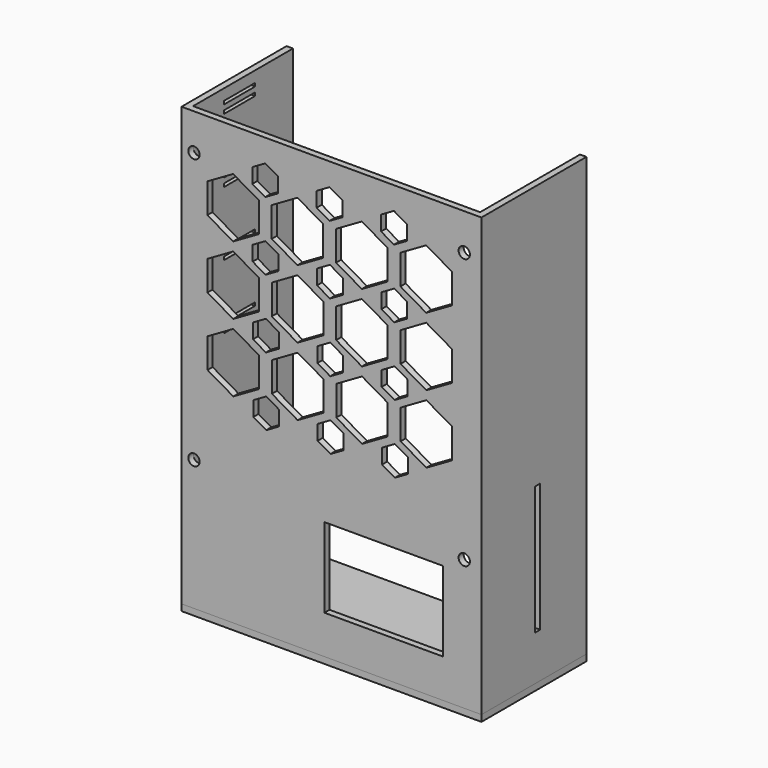
from build123d import *

# Parameters (mm, degrees)
F1_DEPTH  = 170
F2_W      = 116.5
F2_H      = 2.5
F3_DEPTH  = 51
F4_W      = 46
F4_H      = 31
F5_DEPTH  = 10
F7_DEPTH  = 25
F9_D      = 11
F9_DEPTH  = 38.5365562692
F11_DEPTH = 25
F13_D     = 4.4
F14_W     = 15
F14_H     = 1.25
F15_DEPTH = 51
F16_W     = 2.5
F16_H     = 50
F17_DEPTH = 80


# Not quite as in the source:
# - a feature names something its author has since deleted; it is built from what else it names


with BuildPart() as f1:
    # F0 (on Top) → F1 (new body)
    with BuildSketch(Plane.XY):
        Polygon((-38.5355562692, 51), (-38.5355562692, 0), (77.9644437308, 0), (77.9644437308, 51), (75.4644437308, 51), (75.4644437308, 2.4839404983), (-36.0355562692, 2.4839404983), (-36.0355562692, 51), align=None)
    extrude(amount=F1_DEPTH)

    # F4 (on Front) → F5 (cut)
    with BuildSketch(Plane.XZ):
        with Locations((39.9644437308, 30.5)):
            Rectangle(F4_W, F4_H)
    extrude(amount=-F5_DEPTH, mode=Mode.SUBTRACT)

    # F6 (on Front) → F7 (cut)
    with BuildSketch(Plane.XZ):
        Polygon((21.5, 136.2), (31.5, 130.4264973081), (41.5, 136.2), (41.5, 147.7470053838), (31.5, 153.5205080757), (21.5, 147.7470053838), align=None)
        Polygon((25.8301270189, 145.2470053838), (31.5, 148.5205080757), (37.1698729811, 145.2470053838), (37.1698729811, 138.7), (31.5, 135.4264973081), (25.8301270189, 138.7), align=None, mode=Mode.SUBTRACT)
        Polygon((56.5355562692, 127.0410161514), (46.5355562692, 121.2675134595), (46.5355562692, 109.7205080757), (56.5355562692, 103.9470053838), (66.5355562692, 109.7205080757), (66.5355562692, 121.2675134595), align=None)
        Polygon((56.5355562692, 108.9470053838), (50.8656832881, 112.2205080757), (50.8656832881, 118.7675134595), (56.5355562692, 122.0410161514), (62.2054292503, 118.7675134595), (62.2054292503, 112.2205080757), align=None, mode=Mode.SUBTRACT)
        Polygon((-3.4644437308, 121.2675134595), (-3.4644437308, 109.7205080757), (6.5355562692, 103.9470053838), (16.5355562692, 109.7205080757), (16.5355562692, 121.2675134595), (6.5355562692, 127.0410161514), align=None)
        Polygon((6.5355562692, 122.0410161514), (12.2054292503, 118.7675134595), (12.2054292503, 112.2205080757), (6.5355562692, 108.9470053838), (0.8656832881, 112.2205080757), (0.8656832881, 118.7675134595), align=None, mode=Mode.SUBTRACT)
        Polygon((21.5711125384, 83.2410161514), (31.5711125384, 77.4675134595), (41.5711125384, 83.2410161514), (41.5711125384, 94.7880215352), (31.5711125384, 100.5615242271), (21.5711125384, 94.7880215352), align=None)
        Polygon((25.9012395573, 92.2880215352), (31.5711125384, 95.5615242271), (37.2409855194, 92.2880215352), (37.2409855194, 85.7410161514), (31.5711125384, 82.4675134595), (25.9012395573, 85.7410161514), align=None, mode=Mode.SUBTRACT)
        Polygon((21.5355562692, 109.7205080757), (31.5355562692, 103.9470053838), (41.5355562692, 109.7205080757), (41.5355562692, 121.2675134595), (31.5355562692, 127.0410161514), (21.5355562692, 121.2675134595), align=None)
        Polygon((25.8656832881, 118.7675134595), (31.5355562692, 122.0410161514), (37.2054292503, 118.7675134595), (37.2054292503, 112.2205080757), (31.5355562692, 108.9470053838), (25.8656832881, 112.2205080757), align=None, mode=Mode.SUBTRACT)
        Polygon((-28.5, 147.7470053838), (-28.5, 136.2), (-18.5, 130.4264973081), (-8.5, 136.2), (-8.5, 147.7470053838), (-18.5, 153.5205080757), align=None)
        Polygon((-18.5, 135.4264973081), (-24.1698729811, 138.7), (-24.1698729811, 145.2470053838), (-18.5, 148.5205080757), (-12.8301270189, 145.2470053838), (-12.8301270189, 138.7), align=None, mode=Mode.SUBTRACT)
        Polygon((-28.4644437308, 121.2675134595), (-28.4644437308, 109.7205080757), (-18.4644437308, 103.9470053838), (-8.4644437308, 109.7205080757), (-8.4644437308, 121.2675134595), (-18.4644437308, 127.0410161514), align=None)
        Polygon((-18.4644437308, 108.9470053838), (-24.1343167119, 112.2205080757), (-24.1343167119, 118.7675134595), (-18.4644437308, 122.0410161514), (-12.7945707497, 118.7675134595), (-12.7945707497, 112.2205080757), align=None, mode=Mode.SUBTRACT)
        Polygon((-28.4288874616, 94.7880215352), (-28.4288874616, 83.2410161514), (-18.4288874616, 77.4675134595), (-8.4288874616, 83.2410161514), (-8.4288874616, 94.7880215352), (-18.4288874616, 100.5615242271), align=None)
        Polygon((-18.4288874616, 82.4675134595), (-24.0987604427, 85.7410161514), (-24.0987604427, 92.2880215352), (-18.4288874616, 95.5615242271), (-12.7590144806, 92.2880215352), (-12.7590144806, 85.7410161514), align=None, mode=Mode.SUBTRACT)
        Polygon((-3.4288874616, 94.7880215352), (-3.4288874616, 83.2410161514), (6.5711125384, 77.4675134595), (16.5711125384, 83.2410161514), (16.5711125384, 94.7880215352), (6.5711125384, 100.5615242271), align=None)
        Polygon((6.5711125384, 95.5615242271), (12.2409855194, 92.2880215352), (12.2409855194, 85.7410161514), (6.5711125384, 82.4675134595), (0.9012395573, 85.7410161514), (0.9012395573, 92.2880215352), align=None, mode=Mode.SUBTRACT)
        Polygon((56.5711125384, 100.5615242271), (46.5711125384, 94.7880215352), (46.5711125384, 83.2410161514), (56.5711125384, 77.4675134595), (66.5711125384, 83.2410161514), (66.5711125384, 94.7880215352), align=None)
        Polygon((56.5711125384, 82.4675134595), (50.9012395573, 85.7410161514), (50.9012395573, 92.2880215352), (56.5711125384, 95.5615242271), (62.2409855194, 92.2880215352), (62.2409855194, 85.7410161514), align=None, mode=Mode.SUBTRACT)
        Polygon((56.5, 153.5205080757), (46.5, 147.7470053838), (46.5, 136.2), (56.5, 130.4264973081), (66.5, 136.2), (66.5, 147.7470053838), align=None)
        Polygon((56.5, 135.4264973081), (50.8301270189, 138.7), (50.8301270189, 145.2470053838), (56.5, 148.5205080757), (62.1698729811, 145.2470053838), (62.1698729811, 138.7), align=None, mode=Mode.SUBTRACT)
        Polygon((-3.5, 147.7470053838), (-3.5, 136.2), (6.5, 130.4264973081), (16.5, 136.2), (16.5, 147.7470053838), (6.5, 153.5205080757), align=None)
        Polygon((6.5, 148.5205080757), (12.1698729811, 145.2470053838), (12.1698729811, 138.7), (6.5, 135.4264973081), (0.8301270189, 138.7), (0.8301270189, 145.2470053838), align=None, mode=Mode.SUBTRACT)
        Polygon((50.8301270189, 145.2470053838), (50.8301270189, 138.7), (56.5, 135.4264973081), (62.1698729811, 138.7), (62.1698729811, 145.2470053838), (56.5, 148.5205080757), align=None)
        Polygon((37.1698729811, 145.2470053838), (31.5, 148.5205080757), (25.8301270189, 145.2470053838), (25.8301270189, 138.7), (31.5, 135.4264973081), (37.1698729811, 138.7), align=None)
        Polygon((12.1698729811, 138.7), (12.1698729811, 145.2470053838), (6.5, 148.5205080757), (0.8301270189, 145.2470053838), (0.8301270189, 138.7), (6.5, 135.4264973081), align=None)
        Polygon((-24.1698729811, 145.2470053838), (-24.1698729811, 138.7), (-18.5, 135.4264973081), (-12.8301270189, 138.7), (-12.8301270189, 145.2470053838), (-18.5, 148.5205080757), align=None)
        Polygon((-24.1343167119, 118.7675134595), (-24.1343167119, 112.2205080757), (-18.4644437308, 108.9470053838), (-12.7945707497, 112.2205080757), (-12.7945707497, 118.7675134595), (-18.4644437308, 122.0410161514), align=None)
        Polygon((12.2054292503, 112.2205080757), (12.2054292503, 118.7675134595), (6.5355562692, 122.0410161514), (0.8656832881, 118.7675134595), (0.8656832881, 112.2205080757), (6.5355562692, 108.9470053838), align=None)
        Polygon((37.2054292503, 118.7675134595), (31.5355562692, 122.0410161514), (25.8656832881, 118.7675134595), (25.8656832881, 112.2205080757), (31.5355562692, 108.9470053838), (37.2054292503, 112.2205080757), align=None)
        Polygon((50.8656832881, 118.7675134595), (50.8656832881, 112.2205080757), (56.5355562692, 108.9470053838), (62.2054292503, 112.2205080757), (62.2054292503, 118.7675134595), (56.5355562692, 122.0410161514), align=None)
        Polygon((50.9012395573, 92.2880215352), (50.9012395573, 85.7410161514), (56.5711125384, 82.4675134595), (62.2409855194, 85.7410161514), (62.2409855194, 92.2880215352), (56.5711125384, 95.5615242271), align=None)
        Polygon((37.2409855194, 92.2880215352), (31.5711125384, 95.5615242271), (25.9012395573, 92.2880215352), (25.9012395573, 85.7410161514), (31.5711125384, 82.4675134595), (37.2409855194, 85.7410161514), align=None)
        Polygon((12.2409855194, 85.7410161514), (12.2409855194, 92.2880215352), (6.5711125384, 95.5615242271), (0.9012395573, 92.2880215352), (0.9012395573, 85.7410161514), (6.5711125384, 82.4675134595), align=None)
        Polygon((-24.0987604427, 92.2880215352), (-24.0987604427, 85.7410161514), (-18.4288874616, 82.4675134595), (-12.7590144806, 85.7410161514), (-12.7590144806, 92.2880215352), (-18.4288874616, 95.5615242271), align=None)
    extrude(amount=-F7_DEPTH, mode=Mode.SUBTRACT)

    # F9 (through all, one way)
    with BuildSketch(Plane.YZ):
        with Locations((51, 7.0211063139)):
            Circle(F9_D / 2)
    extrude(amount=-F9_DEPTH, mode=Mode.SUBTRACT)

    # F10 (on Front) → F11 (cut)
    with BuildSketch(Plane.XZ):
        Polygon((-6.0300837602, 149.6529683063), (-1.0300837602, 152.5397196522), (-1.0300837602, 158.3132223441), (-6.0300837602, 161.19997369), (-11.0300837602, 158.3132223441), (-11.0300837602, 152.5397196522), align=None)
        Polygon((13.9699162398, 152.5397196522), (18.9699162398, 149.6529683063), (23.9699162398, 152.5397196522), (23.9699162398, 158.3132223441), (18.9699162398, 161.19997369), (13.9699162398, 158.3132223441), align=None)
        Polygon((38.9699162398, 152.5397196522), (43.9699162398, 149.6529683063), (48.9699162398, 152.5397196522), (48.9699162398, 158.3132223441), (43.9699162398, 161.19997369), (38.9699162398, 158.3132223441), align=None)
        Polygon((49.0999997311, 126.0132223441), (49.0999997311, 131.786725036), (44.0999997311, 134.6734763819), (39.0999997311, 131.786725036), (39.0999997311, 126.0132223441), (44.0999997311, 123.1264709981), align=None)
        Polygon((24.0999997311, 126.0132223441), (24.0999997311, 131.786725036), (19.0999997311, 134.6734763819), (14.0999997311, 131.786725036), (14.0999997311, 126.0132223441), (19.0999997311, 123.1264709981), align=None)
        Polygon((-10.9000002689, 126.0132223441), (-5.9000002689, 123.1264709981), (-0.9000002689, 126.0132223441), (-0.9000002689, 131.786725036), (-5.9000002689, 134.6734763819), (-10.9000002689, 131.786725036), align=None)
        Polygon((49.2300832223, 99.486725036), (49.2300832223, 105.2602277279), (44.2300832223, 108.1469790738), (39.2300832223, 105.2602277279), (39.2300832223, 99.486725036), (44.2300832223, 96.59997369), align=None)
        Polygon((24.2300832223, 99.486725036), (24.2300832223, 105.2602277279), (19.2300832223, 108.1469790738), (14.2300832223, 105.2602277279), (14.2300832223, 99.486725036), (19.2300832223, 96.59997369), align=None)
        Polygon((-10.7699167777, 99.486725036), (-5.7699167777, 96.59997369), (-0.7699167777, 99.486725036), (-0.7699167777, 105.2602277279), (-5.7699167777, 108.1469790738), (-10.7699167777, 105.2602277279), align=None)
        Polygon((49.3601667136, 72.9602277279), (49.3601667136, 78.7337304198), (44.3601667136, 81.6204817657), (39.3601667136, 78.7337304198), (39.3601667136, 72.9602277279), (44.3601667136, 70.0734763819), align=None)
        Polygon((24.3601667136, 72.9602277279), (24.3601667136, 78.7337304198), (19.3601667136, 81.6204817657), (14.3601667136, 78.7337304198), (14.3601667136, 72.9602277279), (19.3601667136, 70.0734763819), align=None)
        Polygon((-10.6398332864, 72.9602277279), (-5.6398332864, 70.0734763819), (-0.6398332864, 72.9602277279), (-0.6398332864, 78.7337304198), (-5.6398332864, 81.6204817657), (-10.6398332864, 78.7337304198), align=None)
    extrude(amount=-F11_DEPTH, mode=Mode.SUBTRACT)

    # F13 (through all)
    with Locations(Plane.XZ):
        with Locations((-33.7085053325, 155.8299248969), (71.2914946675, 155.8299248969), (71.2914946675, 50.8299248969), (-33.7085053325, 50.8299248969)):
            Hole(F13_D / 2)

    # F14 (on Right) → F15 (cut)
    with BuildSketch(Plane.YZ):
        with Locations((25.0782795995, 86.8455207348)):
            Rectangle(F14_W, F14_H)
        with Locations((25.0782795995, 90.0845150445)):
            Rectangle(F14_W, F14_H)
        with Locations((25.0782795995, 111.8455207348)):
            Rectangle(F14_W, F14_H)
        with Locations((25.0782795995, 115.0845150445)):
            Rectangle(F14_W, F14_H)
        with Locations((25.0782795995, 136.8455207348)):
            Rectangle(F14_W, F14_H)
        with Locations((25.0782795995, 140.0845150445)):
            Rectangle(F14_W, F14_H)
        with Locations((25.0782795995, 161.8455207348)):
            Rectangle(F14_W, F14_H)
        with Locations((25.0782795995, 165.0845150445)):
            Rectangle(F14_W, F14_H)
    extrude(amount=-F15_DEPTH, mode=Mode.SUBTRACT)

    # F16 (on Right) → F17 (cut)
    with BuildSketch(Plane.YZ):
        with Locations((27.25, 42.4440450315)):
            Rectangle(F16_W, F16_H)
    extrude(amount=F17_DEPTH, mode=Mode.SUBTRACT)


with BuildPart() as f3:
    # F2 (on Front) → F3 (new body)
    with BuildSketch(Plane.XZ):
        with Locations((19.7144437308, -1.25)):
            Rectangle(F2_W, F2_H)
    extrude(amount=-F3_DEPTH)


solid = Compound([f1.part, f3.part])
